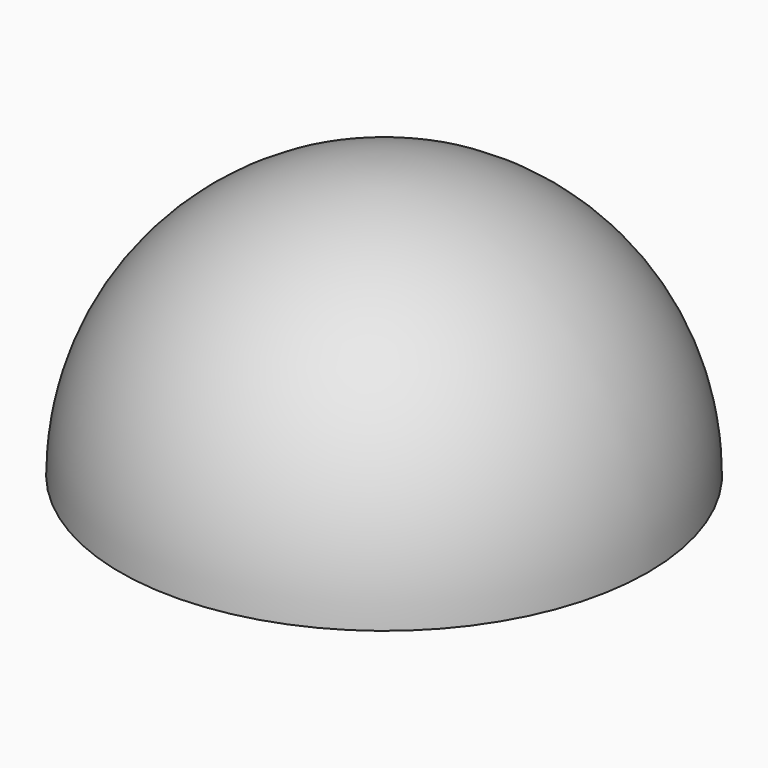
from build123d import *


# Not quite as in the source:
# - the program builds the solid bodies; features that only make, move or delete a surface that nothing else refers to are left out


with BuildPart() as f1:
    # F0 (on Front) → F1 (revolve)
    with BuildSketch(Plane.XZ):
        with BuildLine():
            Line((0, 0), (90, 0))
            ThreePointArc((90, 0), (63.6396103068, 63.6396103068), (0, 90))
            Line((0, 90), (0, 0))
        make_face()
    revolve(axis=Axis((0, 0, 45), (0, 0, 1)))


solid = f1.part
